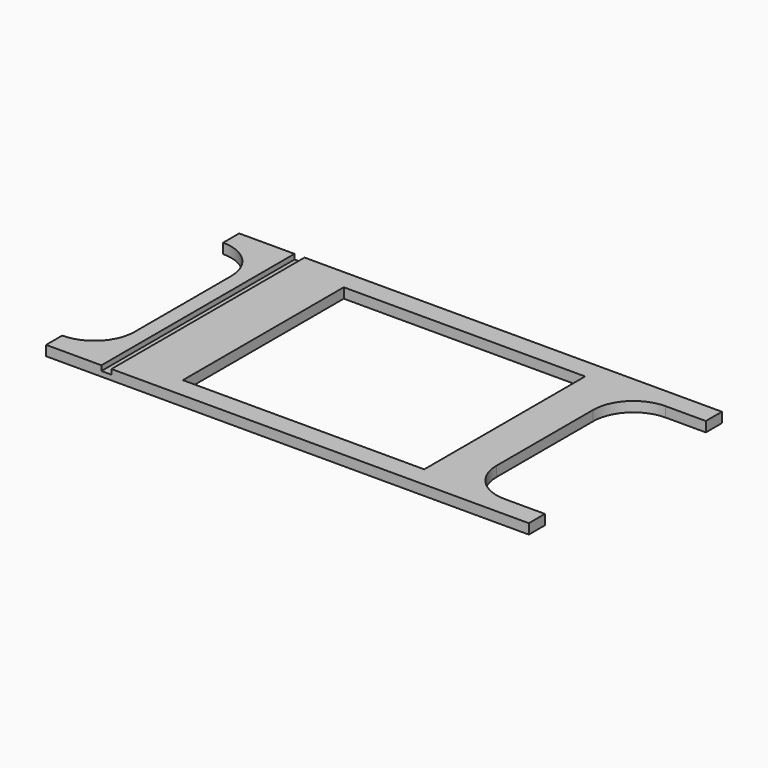
from build123d import *

# Parameters (mm, degrees)
F0_W     = 304.8
F0_H     = 254
F1_DEPTH = 12.7
F2_W     = 12.7
F2_H     = 304.8
F3_DEPTH = 6.35
F4_R     = 50.8
F5_W     = 50.8
F5_H     = 254
F6_DEPTH = 12.7
F7_R     = 50.79999


# Not quite as in the source:
# - a fillet or chamfer is up to 0.001 mm smaller than in the source, because OpenCascade refuses the exact size
# - a feature of the source that left no trace in its solid (it failed there, or was rolled back) is left out


with BuildPart() as f1:
    # F0 (on Top) → F1 (new body)
    with BuildSketch(Plane.XY):
        Polygon((304.8, 127), (304.8, 152.4), (-304.8, 152.4), (-304.8, -152.4), (304.8, -152.4), (304.8, -127), (203.2, -127), (203.2, 127), align=None)
        Rectangle(F0_W, F0_H, mode=Mode.SUBTRACT)
    extrude(amount=F1_DEPTH)

    # F2 (on face) → F3 (cut)
    with BuildSketch(Plane.XY.offset(12.7)):
        with Locations((-228.6, 0)):
            Rectangle(F2_W, F2_H)
    extrude(amount=-F3_DEPTH, mode=Mode.SUBTRACT)

    # F4
    f4_edges = [f1.edges().sort_by_distance(p)[0] for p in [
        (203.2, -127, 6.35),
        (203.2, 127, 6.35),
    ]]
    fillet(f4_edges, radius=F4_R)

    # F5 (on face) → F6 (cut)
    with BuildSketch(Plane.XY.offset(12.7)):
        with Locations((-279.4, 0)):
            Rectangle(F5_W, F5_H)
    extrude(amount=-F6_DEPTH, mode=Mode.SUBTRACT)

    # F7 (radius 50.8 in the source; OpenCascade refuses exactly that, so slightly less here)
    f7_edges = [f1.edges().sort_by_distance(p)[0] for p in [
        (-254, 127, 6.35),
        (-254, -127, 6.35),
    ]]
    fillet(f7_edges, radius=F7_R)


solid = f1.part
